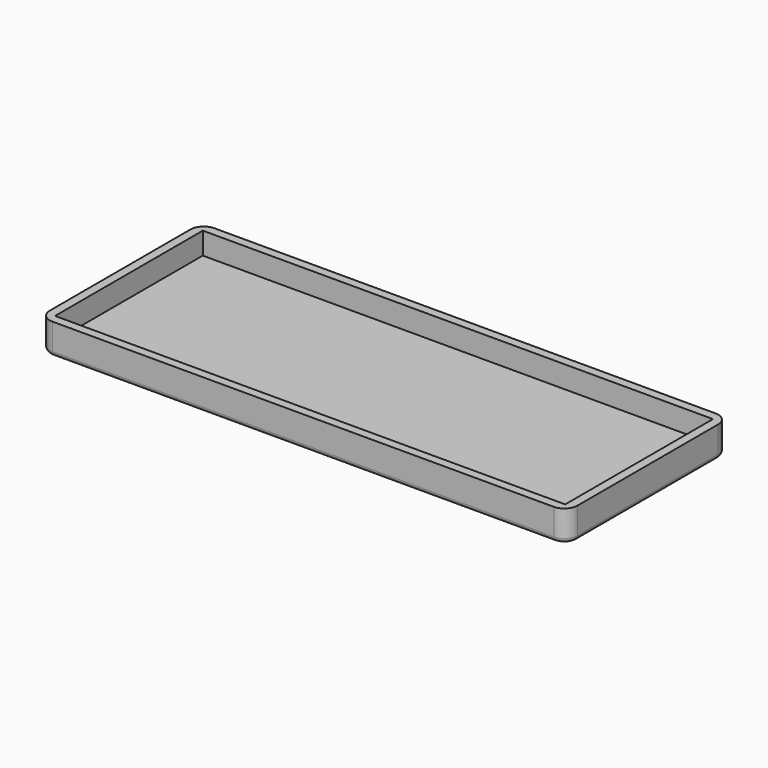
from build123d import *

# Parameters (mm, degrees)
F0_W     = 120
F0_H     = 46
F1_DEPTH = 2
F2_W     = 120
F2_H     = 46
F3_DEPTH = 5
F4_R     = 3
F5_R     = 1
F6_DEPTH = 25


with BuildPart() as f1:
    # F0 (on Top) → F1 (new body)
    with BuildSketch(Plane.XY):
        Rectangle(F0_W, F0_H)
    extrude(amount=F1_DEPTH)

    # F2 (on face) → F3 (join)
    with BuildSketch(Plane.XY.offset(2)):
        Rectangle(F2_W, F2_H)
        Polygon((58, 21), (58, -21), (-57.0000000355, -21), (-58, -21), (-58, -20), (-58, -18), (-58, 21), align=None, mode=Mode.SUBTRACT)
    extrude(amount=F3_DEPTH)

    # F4
    f4_edges = [f1.edges().sort_by_distance(p)[0] for p in [
        (-60, 23, 3.5),
        (-60, -23, 3.5),
        (60, 23, 3.5),
        (60, -23, 3.5),
    ]]
    fillet(f4_edges, radius=F4_R)

    # F5
    f5_edges = [f1.edges().sort_by_distance(p)[0] for p in [
        (0, 23, 0),
        (-59.12132, 22.12132, 0),
        (-60, 0, 0),
        (-59.12132, -22.12132, 0),
        (0, -23, 0),
        (60, 0, 0),
        (59.12132, 22.12132, 0),
        (59.12132, -22.12132, 0),
    ]]
    fillet(f5_edges, radius=F5_R)

    # F2 (on face) → F6 (cut)
    with BuildSketch(Plane.XY.offset(2)):
        with BuildLine():
            ThreePointArc((-56, -18), (-57, -17), (-58, -18))
            ThreePointArc((-58, -18), (-57.7071067812, -18.7071067812), (-57, -19))
            ThreePointArc((-57, -19), (-56.2928932188, -18.7071067812), (-56, -18))
        make_face()
        with BuildLine():
            ThreePointArc((-57, -19), (-56.2928932188, -19.2928932188), (-56, -20))
            Line((-56, -20), (-56, -18))
            ThreePointArc((-56, -18), (-56.2928932188, -18.7071067812), (-57, -19))
        make_face()
        with BuildLine():
            Line((-58, -18), (-58, -20))
            ThreePointArc((-58, -20), (-57.7071067812, -19.2928932188), (-57, -19))
            ThreePointArc((-57, -19), (-57.7071067812, -18.7071067812), (-58, -18))
        make_face()
        with BuildLine():
            ThreePointArc((-58, -20), (-57.7071067937, -20.7071067687), (-57.0000000355, -21))
            ThreePointArc((-57.0000000355, -21), (-56.2928932313, -20.7071067937), (-56, -20))
            ThreePointArc((-56, -20), (-56.2928932188, -19.2928932188), (-57, -19))
            ThreePointArc((-57, -19), (-57.7071067812, -19.2928932188), (-58, -20))
        make_face()
    extrude(amount=-F6_DEPTH, mode=Mode.SUBTRACT)


solid = f1.part
